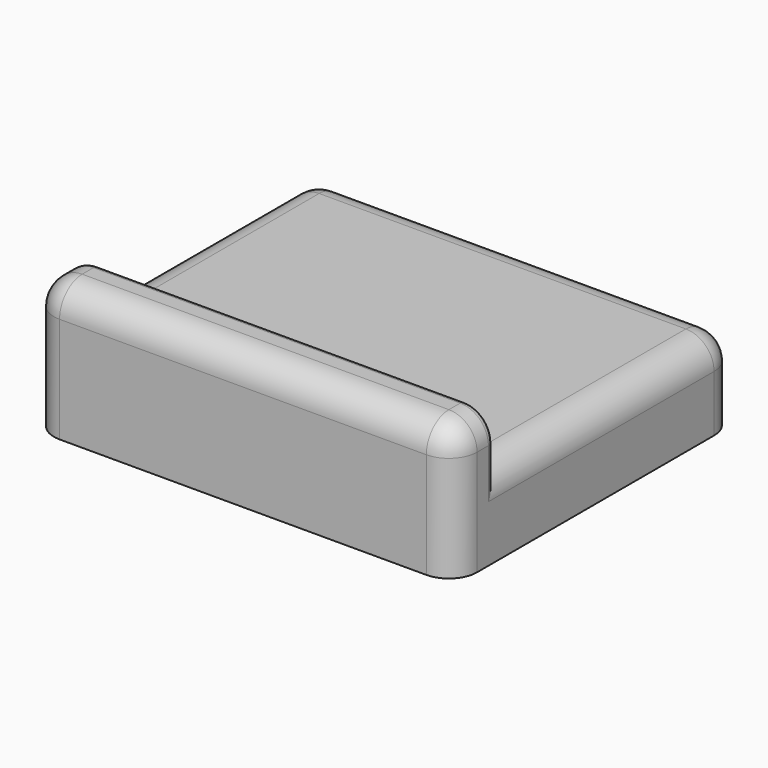
from build123d import *

# Parameters (mm, degrees)
F0_W         = 76.2
F0_H         = 63.5
F1_DEPTH     = 15.24
F2_W         = 76.2
F2_H         = 8.89
F3_DEPTH     = 8.89
F4_R         = 5.08
F5_T1_DEPTH  = 16.51
F5_T3_DEPTH  = 49.53
F5_T5_DEPTH  = 66.04
F5_T7_DEPTH  = 22.86
F5_S11_W     = 5.08
F5_S11_H     = 5.08
F5_T12_DEPTH = 5.08
F5_S17_W     = 5.08
F5_S17_H     = 5.08
F5_T18_DEPTH = 5.08
F5_S23_W     = 5.08
F5_S23_H     = 5.08
F5_T24_DEPTH = 5.08
F5_S29_W     = 5.08
F5_S29_H     = 5.08
F5_T30_DEPTH = 5.08
F6_R         = 1.27


# Not quite as in the source:
# - a fillet or chamfer that OpenCascade refuses, or shapes differently, is made with other operations: its cross-section is extruded or revolved along the edge and cut away or added


with BuildPart() as f1:
    # F0 (on Top) → F1 (new body)
    with BuildSketch(Plane.XY):
        Rectangle(F0_W, F0_H)
    extrude(amount=F1_DEPTH)

    # F2 (on face) → F3 (join)
    with BuildSketch(Plane.XY.offset(15.24)):
        with Locations((0, -27.305)):
            Rectangle(F2_W, F2_H)
    extrude(amount=F3_DEPTH)

    # F4
    f4_edges = [f1.edges().sort_by_distance(p)[0] for p in [
        (38.1, -31.75, 12.065),
        (-38.1, -31.75, 12.065),
        (0, -31.75, 24.13),
    ]]
    fillet(f4_edges, radius=F4_R)

    # F5: fillet of radius 5.08 on 7 edges, made by hand

    # F5_s2 → F5_t1 (cut)
    with BuildSketch(Plane.XZ.offset(10.16)):
        with BuildLine():
            ThreePointArc((-33.02, 24.13), (-36.6121024484, 22.6421024484), (-38.1, 19.05))
            Line((-38.1, 19.05), (-38.1, 24.13))
            Line((-38.1, 24.13), (-33.02, 24.13))
        make_face()
        with BuildLine():
            ThreePointArc((38.1, 19.05), (36.6121024484, 22.6421024484), (33.02, 24.13))
            Line((33.02, 24.13), (38.1, 24.13))
            Line((38.1, 24.13), (38.1, 19.05))
        make_face()
    extrude(amount=F5_T1_DEPTH, mode=Mode.SUBTRACT)

    # F5_s4 → F5_t3 (cut)
    with BuildSketch(Plane.XZ.offset(-26.67)):
        with BuildLine():
            ThreePointArc((-33.02, 15.24), (-36.6121024484, 13.7521024484), (-38.1, 10.16))
            Line((-38.1, 10.16), (-38.1, 15.24))
            Line((-38.1, 15.24), (-33.02, 15.24))
        make_face()
        with BuildLine():
            ThreePointArc((38.1, 10.16), (36.6121024484, 13.7521024484), (33.02, 15.24))
            Line((33.02, 15.24), (38.1, 15.24))
            Line((38.1, 15.24), (38.1, 10.16))
        make_face()
    extrude(amount=F5_T3_DEPTH, mode=Mode.SUBTRACT)

    # F5_s6 → F5_t5 (cut)
    with BuildSketch(Plane.YZ.offset(-33.02)):
        with BuildLine():
            ThreePointArc((26.67, 15.24), (30.2621024484, 13.7521024484), (31.75, 10.16))
            Line((31.75, 10.16), (31.75, 15.24))
            Line((31.75, 15.24), (26.67, 15.24))
        make_face()
    extrude(amount=F5_T5_DEPTH, mode=Mode.SUBTRACT)

    # F5_s8 → F5_t7 (cut)
    with BuildSketch(Plane.XY.offset(-12.7)):
        with BuildLine():
            ThreePointArc((38.1, 26.67), (36.6121024484, 30.2621024484), (33.02, 31.75))
            Line((33.02, 31.75), (38.1, 31.75))
            Line((38.1, 31.75), (38.1, 26.67))
        make_face()
        with BuildLine():
            ThreePointArc((-33.02, 31.75), (-36.6121024484, 30.2621024484), (-38.1, 26.67))
            Line((-38.1, 26.67), (-38.1, 31.75))
            Line((-38.1, 31.75), (-33.02, 31.75))
        make_face()
    extrude(amount=F5_T7_DEPTH, mode=Mode.SUBTRACT)


with BuildPart() as f5_tool10:
    # F5_s11 → F5_t12 (new body)
    with BuildSketch(Plane.YZ.offset(33.02)):
        with Locations((-29.21, 21.59)):
            Rectangle(F5_S11_W, F5_S11_H)
    extrude(amount=F5_T12_DEPTH)

    # F5_s13 → F5_t14 (revolve, cut)
    with BuildSketch(Plane(origin=(33.02, -26.67, 19.05), x_dir=(0, 0.7071067812, -0.7071067812), z_dir=(0, -0.7071067812, -0.7071067812))):
        with BuildLine():
            ThreePointArc((0, -5.08), (5.08, 0), (0, 5.08))
            Line((0, 5.08), (0, -5.08))
        make_face()
    revolve(axis=Axis((33.02, -26.67, 19.05), (1, 0, 0)), mode=Mode.SUBTRACT)


with BuildPart() as f1_1:
    add(f1.part)

    # F5_t9: cut F5_tool10
    add(f5_tool10.part, mode=Mode.SUBTRACT)


with BuildPart() as f5_tool16:
    # F5_s17 → F5_t18 (new body)
    with BuildSketch(Plane.XY.offset(19.05)):
        with Locations((-35.56, -29.21)):
            Rectangle(F5_S17_W, F5_S17_H)
    extrude(amount=F5_T18_DEPTH)

    # F5_s19 → F5_t20 (revolve, cut)
    with BuildSketch(Plane(origin=(-33.02, -26.67, 19.05), x_dir=(0.7071067812, 0.7071067812, 0), z_dir=(0.7071067812, -0.7071067812, 0))):
        with BuildLine():
            ThreePointArc((0, -5.08), (5.08, 0), (0, 5.08))
            Line((0, 5.08), (0, -5.08))
        make_face()
    revolve(axis=Axis((-33.02, -26.67, 19.05), (0, 0, 1)), mode=Mode.SUBTRACT)


with BuildPart() as f1_2:
    add(f1_1.part)

    # F5_t15: cut F5_tool16
    add(f5_tool16.part, mode=Mode.SUBTRACT)


with BuildPart() as f5_tool22:
    # F5_s23 → F5_t24 (new body)
    with BuildSketch(Plane.XY.offset(10.16)):
        with Locations((-35.56, 29.21)):
            Rectangle(F5_S23_W, F5_S23_H)
    extrude(amount=F5_T24_DEPTH)

    # F5_s25 → F5_t26 (revolve, cut)
    with BuildSketch(Plane(origin=(-33.02, 26.67, 10.16), x_dir=(0.7071067812, -0.7071067812, 0), z_dir=(-0.7071067812, -0.7071067812, 0))):
        with BuildLine():
            ThreePointArc((0, -5.08), (5.08, 0), (0, 5.08))
            Line((0, 5.08), (0, -5.08))
        make_face()
    revolve(axis=Axis((-33.02, 26.67, 10.16), (0, 0, 1)), mode=Mode.SUBTRACT)


with BuildPart() as f1_3:
    add(f1_2.part)

    # F5_t21: cut F5_tool22
    add(f5_tool22.part, mode=Mode.SUBTRACT)


with BuildPart() as f5_tool28:
    # F5_s29 → F5_t30 (new body)
    with BuildSketch(Plane.YZ.offset(33.02)):
        with Locations((29.21, 12.7)):
            Rectangle(F5_S29_W, F5_S29_H)
    extrude(amount=F5_T30_DEPTH)

    # F5_s31 → F5_t32 (revolve, cut)
    with BuildSketch(Plane(origin=(33.02, 26.67, 10.16), x_dir=(0, -0.7071067812, -0.7071067812), z_dir=(0, -0.7071067812, 0.7071067812))):
        with BuildLine():
            ThreePointArc((0, -5.08), (5.08, 0), (0, 5.08))
            Line((0, 5.08), (0, -5.08))
        make_face()
    revolve(axis=Axis((33.02, 26.67, 10.16), (1, 0, 0)), mode=Mode.SUBTRACT)


with BuildPart() as f1_4:
    add(f1_3.part)

    # F5_t27: cut F5_tool28
    add(f5_tool28.part, mode=Mode.SUBTRACT)

    # F6
    f6_edges = [f1_4.edges().sort_by_distance(p)[0] for p in [
        (38.1, -22.86, 14.605),
        (36.612102, -22.86, 22.642102),
        (-38.1, -22.86, 14.605),
        (-36.612102, -22.86, 22.642102),
        (0, -22.86, 24.13),
    ]]
    fillet(f6_edges, radius=F6_R)


solid = f1_4.part
